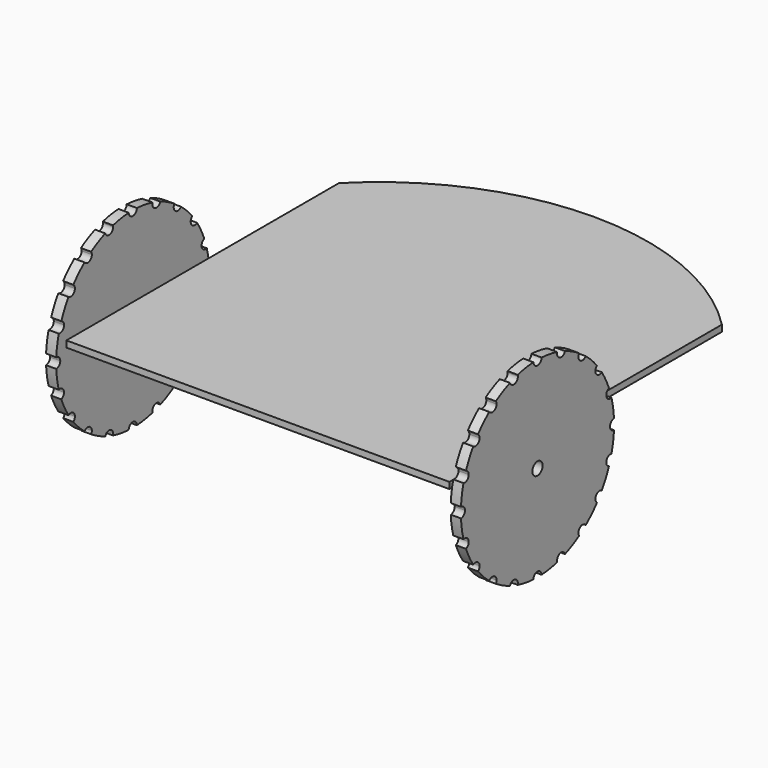
from build123d import *

# Parameters (mm, degrees)
F0_R      = 120
F1_DEPTH  = 5
F2_DEPTH  = 5
F4_R      = 5
F5_DEPTH  = 8
F10_R     = 5
F11_DEPTH = 25


# Not quite as in the source:
# - ends of sketch curves that miss each other by under 0.0002 mm in the source are joined


with BuildPart() as f1:
    # F0 (on Top) → F1 (new body)
    with BuildSketch(Plane.XY):
        Circle(F0_R)
    extrude(amount=F1_DEPTH)

    # F10 (on face) → F11 (cut)
    with BuildSketch(Plane.YZ.offset(163)):
        with Locations((-70, 0)):
            Circle(F10_R)
    extrude(amount=-F11_DEPTH, mode=Mode.SUBTRACT)


with BuildPart() as f2:
    # F0 (on Top) → F2 (new body)
    with BuildSketch(Plane.XY):
        with BuildLine():
            ThreePointArc((150, 126.832395792), (0, 189.4341861589), (-150, 126.832395792))
            Line((-150, 126.832395792), (150, 126.832395792))
        make_face()
        Polygon((150, 126.832395792), (-150, 126.832395792), (-150, -139.999999998), (150.0000089212, -139.999999998), align=None)
        Circle(F0_R, mode=Mode.SUBTRACT)
        Circle(F0_R)
    extrude(amount=F2_DEPTH)


with BuildPart() as f2_1:
    # F3: moved
    add(f2.part.moved(Location((0, 0, 10))))


with BuildPart() as f5:
    # F4 (on Right) → F5 (new body)
    with BuildSketch(Plane.YZ):
        with BuildLine():
            ThreePointArc((74.8933333333, -3.9985775248), (71, 0), (74.8933333333, 3.9985775248))
            ThreePointArc((74.8933333333, 3.9985775248), (74.0766255446, 11.732584878), (72.4634211022, 19.3404395545))
            ThreePointArc((72.4634211022, 19.3404395545), (67.525012657, 21.9402066006), (69.9921642852, 26.9461859763))
            ThreePointArc((69.9921642852, 26.9461859763), (66.8254893141, 34.0492874805), (62.9402843313, 40.7862796574))
            ThreePointArc((62.9402843313, 40.7862796574), (57.4402066006, 41.7327529128), (58.2396745328, 47.2561139993))
            ThreePointArc((58.2396745328, 47.2561139993), (53.033008589, 53.033008589), (47.2561139993, 58.2396745328))
            ThreePointArc((47.2561139993, 58.2396745328), (41.7327529128, 57.4402066006), (40.7862796574, 62.9402843313))
            ThreePointArc((40.7862796574, 62.9402843313), (34.0492874805, 66.8254893141), (26.9461859763, 69.9921642852))
            ThreePointArc((26.9461859763, 69.9921642852), (21.9402066006, 67.525012657), (19.3404395545, 72.4634211022))
            ThreePointArc((19.3404395545, 72.4634211022), (11.732584878, 74.0766255446), (3.9985775248, 74.8933333333))
            ThreePointArc((3.9985775248, 74.8933333333), (0, 71), (-3.9985775248, 74.8933333333))
            ThreePointArc((-3.9985775248, 74.8933333333), (-11.732584878, 74.0766255446), (-19.3404395545, 72.4634211022))
            ThreePointArc((-19.3404395545, 72.4634211022), (-19.2175285586, 71.9022395535), (-19.1762745781, 71.3292387221))
            ThreePointArc((-19.1762745781, 71.3292387221), (-22.4979109561, 67.3871805292), (-26.9461859763, 69.9921642852))
            ThreePointArc((-26.9461859763, 69.9921642852), (-34.0492874805, 66.8254893141), (-40.7862796574, 62.9402843313))
            ThreePointArc((-40.7862796574, 62.9402843313), (-40.2635237136, 61.8615051342), (-40.0838939219, 60.6762745781))
            ThreePointArc((-40.0838939219, 60.6762745781), (-42.7972083173, 56.8888691133), (-47.2561139993, 58.2396745328))
            ThreePointArc((-47.2561139993, 58.2396745328), (-53.033008589, 53.033008589), (-58.2396745328, 47.2561139993))
            ThreePointArc((-58.2396745328, 47.2561139993), (-57.0883503745, 45.8521698929), (-56.6762745781, 44.0838939219))
            ThreePointArc((-56.6762745781, 44.0838939219), (-58.8129494606, 40.5443996775), (-62.9402843313, 40.7862796574))
            ThreePointArc((-62.9402843313, 40.7862796574), (-66.8254893141, 34.0492874805), (-69.9921642852, 26.9461859763))
            ThreePointArc((-69.9921642852, 26.9461859763), (-68.0621071249, 25.484055141), (-67.3292387221, 23.1762745781))
            ThreePointArc((-67.3292387221, 23.1762745781), (-68.9351553402, 19.9718456492), (-72.4634211022, 19.3404395545))
            ThreePointArc((-72.4634211022, 19.3404395545), (-74.0766255446, 11.732584878), (-74.8933333333, 3.9985775248))
            ThreePointArc((-74.8933333333, 3.9985775248), (-72.134108632, 2.7904599382), (-71, 0))
            ThreePointArc((-71, 0), (-72.134108632, -2.7904599382), (-74.8933333333, -3.9985775248))
            ThreePointArc((-74.8933333333, -3.9985775248), (-74.0766255446, -11.732584878), (-72.4634211022, -19.3404395545))
            ThreePointArc((-72.4634211022, -19.3404395545), (-68.9351553402, -19.9718456492), (-67.3292387221, -23.1762745781))
            ThreePointArc((-67.3292387221, -23.1762745781), (-68.0621071249, -25.484055141), (-69.9921642852, -26.9461859763))
            ThreePointArc((-69.9921642852, -26.9461859763), (-66.8254893141, -34.0492874805), (-62.9402843313, -40.7862796574))
            ThreePointArc((-62.9402843313, -40.7862796574), (-58.8129494606, -40.5443996775), (-56.6762745781, -44.0838939219))
            ThreePointArc((-56.6762745781, -44.0838939219), (-57.0883503745, -45.8521698929), (-58.2396745328, -47.2561139993))
            ThreePointArc((-58.2396745328, -47.2561139993), (-53.033008589, -53.033008589), (-47.2561139993, -58.2396745328))
            ThreePointArc((-47.2561139993, -58.2396745328), (-42.7972083173, -56.8888691133), (-40.0838939219, -60.6762745781))
            ThreePointArc((-40.0838939219, -60.6762745781), (-40.2635237136, -61.8615051342), (-40.7862796574, -62.9402843313))
            ThreePointArc((-40.7862796574, -62.9402843313), (-34.0492874805, -66.8254893141), (-26.9461859763, -69.9921642852))
            ThreePointArc((-26.9461859763, -69.9921642852), (-22.4979109561, -67.3871805292), (-19.1762745781, -71.3292387221))
            ThreePointArc((-19.1762745781, -71.3292387221), (-19.2175285586, -71.9022395535), (-19.3404395545, -72.4634211022))
            ThreePointArc((-19.3404395545, -72.4634211022), (-11.732584878, -74.0766255446), (-3.9985775248, -74.8933333333))
            ThreePointArc((-3.9985775248, -74.8933333333), (0, -71), (3.9985775248, -74.8933333333))
            ThreePointArc((3.9985775248, -74.8933333333), (11.732584878, -74.0766255446), (19.3404395545, -72.4634211022))
            ThreePointArc((19.3404395545, -72.4634211022), (21.9402066006, -67.525012657), (26.9461859763, -69.9921642852))
            ThreePointArc((26.9461859763, -69.9921642852), (34.0492874805, -66.8254893141), (40.7862796574, -62.9402843313))
            ThreePointArc((40.7862796574, -62.9402843313), (41.7327529128, -57.4402066006), (47.2561139993, -58.2396745328))
            ThreePointArc((47.2561139993, -58.2396745328), (53.033008589, -53.033008589), (58.2396745328, -47.2561139993))
            ThreePointArc((58.2396745328, -47.2561139993), (57.4402066006, -41.7327529128), (62.9402843313, -40.7862796574))
            ThreePointArc((62.9402843313, -40.7862796574), (66.8254893141, -34.0492874805), (69.9921642852, -26.9461859763))
            ThreePointArc((69.9921642852, -26.9461859763), (67.525012657, -21.9402066006), (72.4634211022, -19.3404395545))
            ThreePointArc((72.4634211022, -19.3404395545), (74.0766255446, -11.732584878), (74.8933333333, -3.9985775248))
        make_face()
        Circle(F4_R, mode=Mode.SUBTRACT)
    extrude(amount=F5_DEPTH)


with BuildPart() as f5_1:
    # F6: moved
    add(f5.part.moved(Location((155, 0, 0))))


with BuildPart() as f5_2:
    # F7: moved
    add(f5_1.part.moved(Location((0, -70, 0))))


with BuildPart() as f8_1:
    # F8: copy of F5
    add(f5_2.part)


with BuildPart() as f9_1:
    # F9: copy of F5
    add(f5_2.part.moved(Location((-317, 0, 0))))


solid = Compound([f1.part, f2_1.part, f5_2.part, f8_1.part, f9_1.part])
